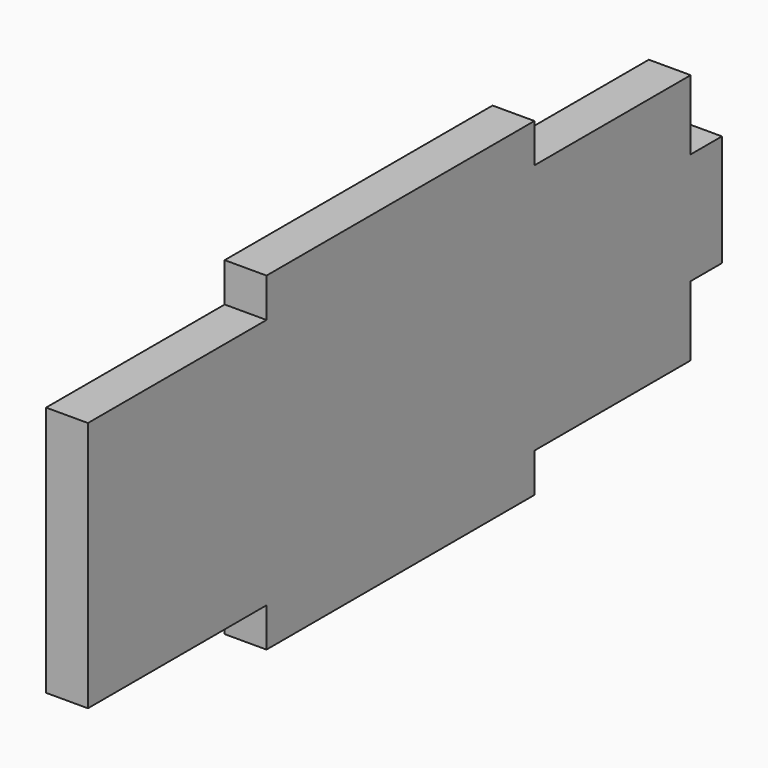
from build123d import *

# Parameters (mm, degrees)
F0_W     = 152.4
F0_H     = 17.78
F0_W_2   = 17.78
F0_H_2   = 50.8
F1_DEPTH = 19.05


# Not quite as in the source:
# - a feature names something its author has since deleted; it is built from what else it names


with BuildPart() as f1:
    # F0 (on Right) → F1 (new body)
    with BuildSketch(Plane.YZ):
        Polygon((-69.85, 0), (-171.45, 0), (-171.45, -114.3), (-69.85, -114.3), (82.55, -114.3), (171.45, -114.3), (171.45, -82.55), (171.45, -31.75), (171.45, 0), (82.55, 0), align=None)
        with Locations((6.35, -123.19)):
            Rectangle(F0_W, F0_H)
        with Locations((180.34, -57.15)):
            Rectangle(F0_W_2, F0_H_2)
        with Locations((6.35, 8.89)):
            Rectangle(F0_W, F0_H)
    extrude(amount=F1_DEPTH)


solid = f1.part
